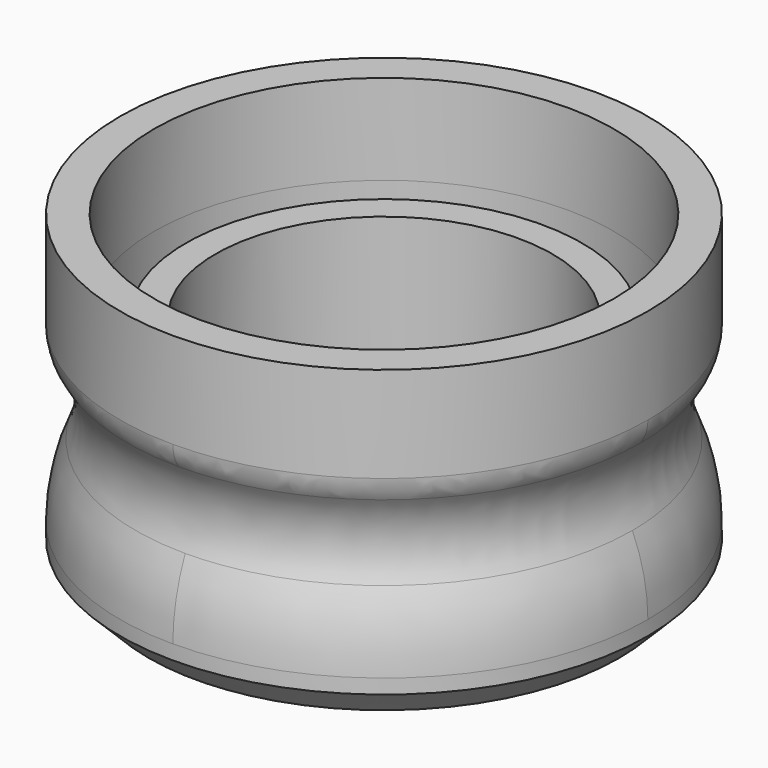
from build123d import *

# Parameters (mm, degrees)
F0_R        = 178.4376232985
F0_R_2      = 155.4455933773
F1_DEPTH    = 100.076
F0_R_3      = 133.9347560768
F0_R_4      = 113.9166344001
F4_DEPTH    = 57.658
F6_T2_ANGLE = 270
F6_T4_ANGLE = 90
F7_R        = 26.1680448885
F8_DEPTH    = 60.96
F9_SIZE     = 5.08


# Not quite as in the source:
# - a fillet or chamfer that OpenCascade refuses, or shapes differently, is made with other operations: its cross-section is extruded or revolved along the edge and cut away or added


with BuildPart() as f1:
    # F0 (on Top) → F1 (new body)
    with BuildSketch(Plane.XY):
        Circle(F0_R)
        Circle(F0_R_2, mode=Mode.SUBTRACT)
    extrude(amount=F1_DEPTH)

    # F2 (on Right) → F3 (revolve, cut)
    with BuildSketch(Plane.YZ):
        with BuildLine():
            Line((-211.7950618267, 10.4418387637), (-179.0756136179, 10.9223620966))
            ThreePointArc((-179.0756136179, 10.9223620966), (-163.2878596781, 49.2948652245), (-179.0756136179, 87.6673683524))
            Line((-179.0756136179, 87.6673683524), (-211.7950618267, 87.6673683524))
            Line((-211.7950618267, 87.6673683524), (-211.7950618267, 10.4418387637))
        make_face()
    revolve(axis=Axis((0, 0, 100.076), (0, 0, 1)), mode=Mode.SUBTRACT)

    # F4 (add): a face of the model
    f4_faces = [f1.faces().sort_by_distance(p)[0] for p in [
        (-173.3906451604, 0, 0),
    ]]
    extrude(f4_faces, amount=F4_DEPTH)

    # F5: chamfer of 25.4 on 1 edges, made by hand

    # F5_s1 → F5_t2 (revolve, cut)
    with BuildSketch(Plane.XZ):
        Polygon((178.4376232985, -32.258), (153.0376232985, -57.658), (178.4376232985, -57.658), align=None)
    revolve(axis=Axis((0, 0, -57.658), (0, 0, 1)), mode=Mode.SUBTRACT)

    # F6: fillet of radius 124.2982132205 on 5 edges, made by hand

    # F6_s1 → F6_t2 (revolve, cut)
    with BuildSketch(Plane.YZ):
        with BuildLine():
            ThreePointArc((-178.4380232985, -22.7388058016), (-175.7769269935, 2.8438127421), (-167.9075785228, 27.3310575799))
            Line((-167.9075785228, 27.3310575799), (-179.2845953673, 32.338043918))
            ThreePointArc((-179.2845953673, 32.338043918), (-182.8167956296, 25.9008324787), (-187.4140893132, 20.1755608169))
            Line((-187.4140893132, 20.1755608169), (-190.8676846206, 11.5773352816))
            ThreePointArc((-190.8676846206, 11.5773352816), (-190.8676846206, -5.58073526), (-190.8680846206, -22.7388058016))
            Line((-190.8680846206, -22.7388058016), (-178.4380232985, -22.7388058016))
        make_face()
    revolve(axis=Axis((0, 0, 11.5773352816), (0, 0, -1)), revolution_arc=F6_T2_ANGLE, mode=Mode.SUBTRACT)

    # F6_s3 → F6_t4 (revolve, cut)
    with BuildSketch(Plane.XZ):
        with BuildLine():
            ThreePointArc((178.4380232985, -22.7388058016), (175.7769269935, 2.8438127421), (167.9075785228, 27.3310575799))
            Line((167.9075785228, 27.3310575799), (179.2845953673, 32.338043918))
            ThreePointArc((179.2845953673, 32.338043918), (182.8167956296, 25.9008324787), (187.4140893132, 20.1755608169))
            Line((187.4140893132, 20.1755608169), (190.8676846206, 11.5773352816))
            ThreePointArc((190.8676846206, 11.5773352816), (190.8676846206, -5.58073526), (190.8680846206, -22.7388058016))
            Line((190.8680846206, -22.7388058016), (178.4380232985, -22.7388058016))
        make_face()
    revolve(axis=Axis((0, 0, 11.5773352816), (0, 0, -1)), revolution_arc=F6_T4_ANGLE, mode=Mode.SUBTRACT)

    # F7
    f7_edges = [f1.edges().sort_by_distance(p)[0] for p in [
        (-118.778106, 118.778106, 27.171632),
        (118.778106, -118.778106, 27.171632),
        (0, -164.10225, 58.683609),
        (126.174453, -126.174453, 87.012395),
        (-126.174453, 126.174453, 87.012395),
    ]]
    fillet(f7_edges, radius=F7_R)

    # F8 (add): a face of the model
    f8_faces = [f1.faces().sort_by_distance(p)[0] for p in [
        (-173.3906451604, 0, 100.076),
    ]]
    extrude(f8_faces, amount=F8_DEPTH)

    # F9
    f9_edges = [f1.edges().sort_by_distance(p)[0] for p in [
        (-155.445593, 0, -55.25003),
    ]]
    chamfer(f9_edges, length=F9_SIZE)


with BuildPart() as f1b:
    # F0 (on Top) → F1, piece 2 (new body)
    with BuildSketch(Plane.XY):
        Circle(F0_R_3)
        Circle(F0_R_4, mode=Mode.SUBTRACT)
    extrude(amount=F1_DEPTH)


solid = Compound([f1.part, f1b.part])
